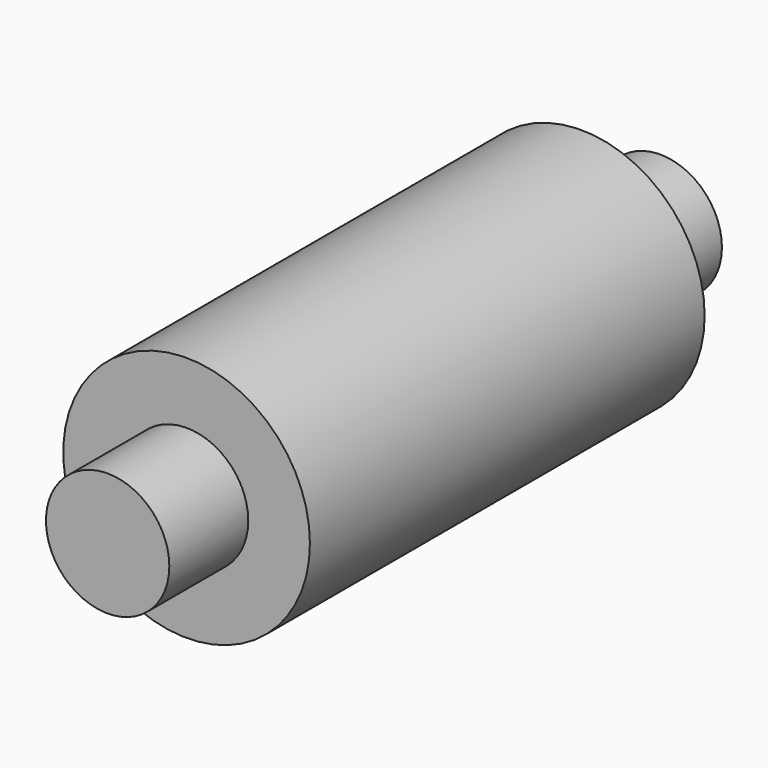
from build123d import *

# Parameters (mm, degrees)
F0_R     = 63.5
F1_DEPTH = 254
F2_R     = 31.75
F3_DEPTH = 50.8


# Not quite as in the source:
# - a pattern or mirror of a feature is missing from the dataset's text; its kind, count and spacing are read off the source's solid


with BuildPart() as f1:
    # F0 (on Front) → F1 (new body)
    with BuildSketch(Plane.XZ):
        Circle(F0_R)
    extrude(amount=F1_DEPTH)

    # F2 (on face) → F3 (join)
    with BuildSketch(Plane.XZ.offset(254)):
        Circle(F2_R)
    f3 = extrude(amount=F3_DEPTH)

    # F3_copies: F3 across plane
    add(f3.mirror(Plane.ZX.offset(-127)))


solid = f1.part
